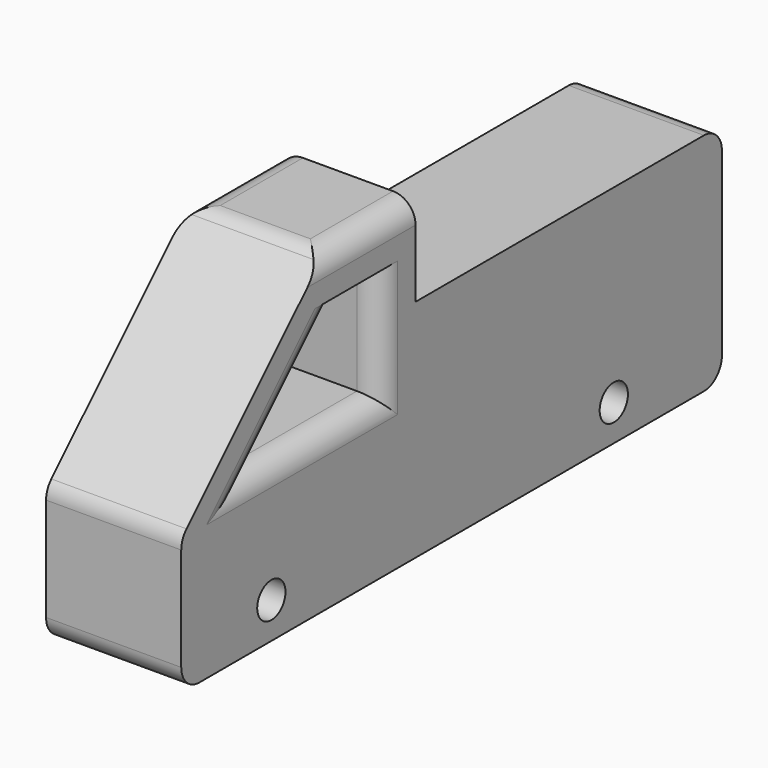
from build123d import *

# Parameters (mm, degrees)
F0_R     = 3.923916639
F1_DEPTH = 15
F2_R     = 5
F2_R_2   = 4.99999


# Not quite as in the source:
# - a fillet or chamfer is up to 0.001 mm smaller than in the source, because OpenCascade refuses the exact size


with BuildPart() as f1:
    # F0 (on Right) → F1 (new body, symmetric)
    with BuildSketch(Plane.YZ):
        Polygon((0, 30), (0, 0), (150, 0), (150, 50), (65, 50), (65, 70), (40, 70), align=None)
        with Locations((25, 8)):
            Circle(F0_R, mode=Mode.SUBTRACT)
        with Locations((120, 8)):
            Circle(F0_R, mode=Mode.SUBTRACT)
        Polygon((44.1421356237, 60), (55, 60), (55, 35), (19.1421356237, 35), align=None, mode=Mode.SUBTRACT)
    extrude(amount=F1_DEPTH, both=True)

    # F2 (call 1 of 7: OpenCascade refuses the feature's edges together)
    f2_edges = [f1.edges().sort_by_distance(p)[0] for p in [
        (15, 52.5, 70),
        (0, 40, 70),
        (-15, 52.5, 70),
    ]]
    fillet(f2_edges, radius=F2_R)

    # F2#2 (call 2 of 7)
    f2_2_edges = [f1.edges().sort_by_distance(p)[0] for p in [
        (0, 0, 30),
    ]]
    fillet(f2_2_edges, radius=F2_R)

    # F2#3 (call 3 of 7)
    f2_3_edges = [f1.edges().sort_by_distance(p)[0] for p in [
        (0, 0, 0),
    ]]
    fillet(f2_3_edges, radius=F2_R)

    # F2#4 (call 4 of 7)
    f2_4_edges = [f1.edges().sort_by_distance(p)[0] for p in [
        (0, 150, 50),
    ]]
    fillet(f2_4_edges, radius=F2_R)

    # F2#5 (call 5 of 7) (radius 5 in the source; OpenCascade refuses exactly that, so slightly less here)
    f2_5_edges = [f1.edges().sort_by_distance(p)[0] for p in [
        (-15, 37.071068, 35),
        (-15, 55, 47.5),
        (-15, 49.571068, 60),
        (-15, 31.642136, 47.5),
    ]]
    fillet(f2_5_edges, radius=F2_R_2)

    # F2#6 (call 6 of 7)
    f2_6_edges = [f1.edges().sort_by_distance(p)[0] for p in [
        (15, 37.071068, 35),
        (15, 55, 47.5),
        (15, 31.642136, 47.5),
    ]]
    fillet(f2_6_edges, radius=F2_R)

    # F2#7 (call 7 of 7)
    f2_7_edges = [f1.edges().sort_by_distance(p)[0] for p in [
        (0, 150, 0),
    ]]
    fillet(f2_7_edges, radius=F2_R)


solid = f1.part
